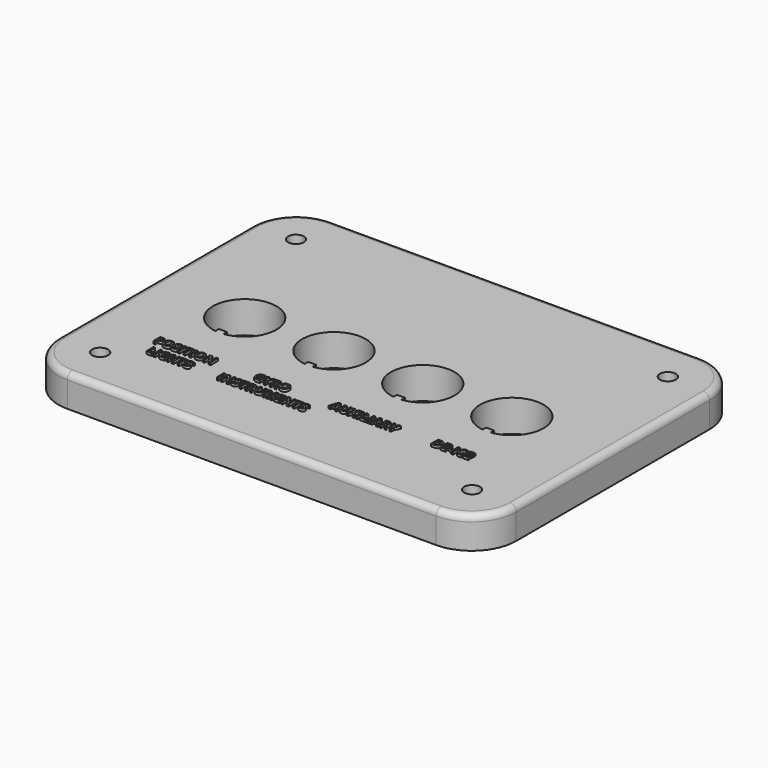
from build123d import *

# Parameters (mm, degrees)
F0_R         = 1.5875
F0_W         = 0.3738893229
F0_H         = 1.7629518229
F0_W_2       = 0.6474574653
F0_H_2       = 0.3013493924
F0_TEXT_SIZE = 2.4694444444
F1_DEPTH     = 6.35
F2_R         = 1.27
F3_DEPTH     = 0.508


# Not quite as in the source:
# - Text() gives the source's letters only with a copy of the font that has no kerning and outlines rounded to 1/6400 em; it was checked with that copy


with BuildPart() as f1:
    # F0 (on Top) → F1 (new body)
    with BuildSketch(Plane.XY):
        with BuildLine():
            ThreePointArc((-45.72, -22.8328104488), (-43.1161792847, -29.1189897335), (-36.83, -31.7228104488))
            Line((-36.83, -31.7228104488), (36.83, -31.7228104488))
            ThreePointArc((36.83, -31.7228104488), (43.1161792847, -29.1189897335), (45.72, -22.8328104488))
            Line((45.72, -22.8328104488), (45.72, 25.4271895512))
            ThreePointArc((45.72, 25.4271895512), (43.1161792847, 31.7133688359), (36.83, 34.3171895512))
            Line((36.83, 34.3171895512), (-36.83, 34.3171895512))
            ThreePointArc((-36.83, 34.3171895512), (-43.1161792847, 31.7133688359), (-45.72, 25.4271895512))
            Line((-45.72, 25.4271895512), (-45.72, -22.8328104488))
        make_face()
        with BuildLine():
            Line((33.655, -28.5478104488), (-33.655, -28.5478104488))
            ThreePointArc((-33.655, -28.5478104488), (-39.9411792847, -25.9439897335), (-42.545, -19.6578104488))
            Line((-42.545, -19.6578104488), (-42.545, 22.2521895512))
            ThreePointArc((-42.545, 22.2521895512), (-39.9411792847, 28.5383688359), (-33.655, 31.1421895512))
            Line((-33.655, 31.1421895512), (33.655, 31.1421895512))
            ThreePointArc((33.655, 31.1421895512), (39.9411792847, 28.5383688359), (42.545, 22.2521895512))
            Line((42.545, 22.2521895512), (42.545, -19.6578104488))
            ThreePointArc((42.545, -19.6578104488), (39.9411792847, -25.9439897335), (33.655, -28.5478104488))
        make_face(mode=Mode.SUBTRACT)
        with BuildLine():
            ThreePointArc((-42.545, -19.6578104488), (-39.9411792847, -25.9439897335), (-33.655, -28.5478104488))
            Line((-33.655, -28.5478104488), (33.655, -28.5478104488))
            ThreePointArc((33.655, -28.5478104488), (39.9411792847, -25.9439897335), (42.545, -19.6578104488))
            Line((42.545, -19.6578104488), (42.545, 22.2521895512))
            ThreePointArc((42.545, 22.2521895512), (39.9411792847, 28.5383688359), (33.655, 31.1421895512))
            Line((33.655, 31.1421895512), (-33.655, 31.1421895512))
            ThreePointArc((-33.655, 31.1421895512), (-39.9411792847, 28.5383688359), (-42.545, 22.2521895512))
            Line((-42.545, 22.2521895512), (-42.545, -19.6578104488))
        make_face()
        with Locations((-37.1475, -23.1503104488)):
            Circle(F0_R, mode=Mode.SUBTRACT)
        Polygon((-30.0736846576, -19.1064444444), (-31.1625553173, -19.1064444444), (-31.1625553173, -17.3434926215), (-30.7886659944, -17.3434926215), (-30.7886659944, -18.7977638889), (-30.0736846576, -18.7977638889), align=None, mode=Mode.SUBTRACT)
        with Locations((-29.5803745447, -18.224968533)):
            Rectangle(F0_W, F0_H, mode=Mode.SUBTRACT)
        with BuildLine():
            Line((-28.2806364805, -18.4277330729), (-28.2806364805, -18.1163515625))
            Line((-28.2806364805, -18.1163515625), (-27.5810891715, -18.1163515625))
            Line((-27.5810891715, -18.1163515625), (-27.5810891715, -19.0304318576))
            add(Edge.make_bspline(
                [(-27.5810891715, -19.0304318576), (-27.7512493277, -19.0859943576), (-27.9013452479, -19.1083736979)],
                knots=[0, 0, 0, 1, 1, 1], degree=2))
            add(Edge.make_bspline(
                [(-27.9013452479, -19.1083736979), (-28.051441168, -19.1307530382), (-28.2080965499, -19.1307530382)],
                knots=[0, 0, 0, 1, 1, 1], degree=2))
            add(Edge.make_bspline(
                [(-28.2080965499, -19.1307530382), (-28.607066168, -19.1307530382), (-28.8175477218, -18.896155816)],
                knots=[0, 0, 0, 1, 1, 1], degree=2))
            add(Edge.make_bspline(
                [(-28.8175477218, -18.896155816), (-29.0280292756, -18.6615585938), (-29.0280292756, -18.2224605035)],
                knots=[0, 0, 0, 1, 1, 1], degree=2))
            add(Edge.make_bspline(
                [(-29.0280292756, -18.2224605035), (-29.0280292756, -17.7957096354), (-28.7837857861, -17.5570609809)],
                knots=[0, 0, 0, 1, 1, 1], degree=2))
            add(Edge.make_bspline(
                [(-28.7837857861, -17.5570609809), (-28.5395422965, -17.3184123264), (-28.107003668, -17.3184123264)],
                knots=[0, 0, 0, 1, 1, 1], degree=2))
            add(Edge.make_bspline(
                [(-28.107003668, -17.3184123264), (-27.8353647791, -17.3184123264), (-27.5834042756, -17.4268363715)],
                knots=[0, 0, 0, 1, 1, 1], degree=2))
            Line((-27.5834042756, -17.4268363715), (-27.7076481993, -17.7258706597))
            add(Edge.make_bspline(
                [(-27.7076481993, -17.7258706597), (-27.9005735465, -17.6294079861), (-28.1093187722, -17.6294079861)],
                knots=[0, 0, 0, 1, 1, 1], degree=2))
            add(Edge.make_bspline(
                [(-28.1093187722, -17.6294079861), (-28.3516330083, -17.6294079861), (-28.4974845708, -17.7922369792)],
                knots=[0, 0, 0, 1, 1, 1], degree=2))
            add(Edge.make_bspline(
                [(-28.4974845708, -17.7922369792), (-28.6433361333, -17.9550659722), (-28.6433361333, -18.2297916667)],
                knots=[0, 0, 0, 1, 1, 1], degree=2))
            add(Edge.make_bspline(
                [(-28.6433361333, -18.2297916667), (-28.6433361333, -18.5168645833), (-28.5258445968, -18.6681180556)],
                knots=[0, 0, 0, 1, 1, 1], degree=2))
            add(Edge.make_bspline(
                [(-28.5258445968, -18.6681180556), (-28.4083530604, -18.8193715278), (-28.1841738069, -18.8193715278)],
                knots=[0, 0, 0, 1, 1, 1], degree=2))
            add(Edge.make_bspline(
                [(-28.1841738069, -18.8193715278), (-28.0668751958, -18.8193715278), (-27.9464897791, -18.7954487847)],
                knots=[0, 0, 0, 1, 1, 1], degree=2))
            Line((-27.9464897791, -18.7954487847), (-27.9464897791, -18.4277330729))
            Line((-27.9464897791, -18.4277330729), (-28.2806364805, -18.4277330729))
        make_face(mode=Mode.SUBTRACT)
        Polygon((-25.7170444666, -17.3434926215), (-25.7170444666, -19.1064444444), (-26.0897762374, -19.1064444444), (-26.0897762374, -18.345546875), (-26.7877801437, -18.345546875), (-26.7877801437, -19.1064444444), (-27.1616694666, -19.1064444444), (-27.1616694666, -17.3434926215), (-26.7877801437, -17.3434926215), (-26.7877801437, -18.0345512153), (-26.0897762374, -18.0345512153), (-26.0897762374, -17.3434926215), align=None, mode=Mode.SUBTRACT)
        Polygon((-24.5919038416, -17.6544882813), (-24.5919038416, -19.1064444444), (-24.9657931645, -19.1064444444), (-24.9657931645, -17.6544882813), (-25.4446338763, -17.6544882813), (-25.4446338763, -17.3434926215), (-24.1134489805, -17.3434926215), (-24.1134489805, -17.6544882813), align=None, mode=Mode.SUBTRACT)
        with BuildLine():
            add(Edge.make_bspline(
                [(-22.8931961593, -18.3256755642), (-22.8015566194, -18.4443246528), (-22.8015566194, -18.6167999132)],
                knots=[0, 0, 0, 1, 1, 1], degree=2))
            add(Edge.make_bspline(
                [(-22.8015566194, -18.6167999132), (-22.8015566194, -18.8556414931), (-22.9734531038, -18.9931972656)],
                knots=[0, 0, 0, 1, 1, 1], degree=2))
            add(Edge.make_bspline(
                [(-22.9734531038, -18.9931972656), (-23.1453495881, -19.1307530382), (-23.4513291888, -19.1307530382)],
                knots=[0, 0, 0, 1, 1, 1], degree=2))
            add(Edge.make_bspline(
                [(-23.4513291888, -19.1307530382), (-23.7337718972, -19.1307530382), (-23.9506199874, -19.0242582465)],
                knots=[0, 0, 0, 1, 1, 1], degree=2))
            Line((-23.9506199874, -19.0242582465), (-23.9506199874, -18.6769926215))
            add(Edge.make_bspline(
                [(-23.9506199874, -18.6769926215), (-23.7723569666, -18.7568637153), (-23.648691819, -18.7892751736)],
                knots=[0, 0, 0, 1, 1, 1], degree=2))
            add(Edge.make_bspline(
                [(-23.648691819, -18.7892751736), (-23.5250266715, -18.8216866319), (-23.4223903868, -18.8216866319)],
                knots=[0, 0, 0, 1, 1, 1], degree=2))
            add(Edge.make_bspline(
                [(-23.4223903868, -18.8216866319), (-23.2996898659, -18.8216866319), (-23.2339023225, -18.7748057726)],
                knots=[0, 0, 0, 1, 1, 1], degree=2))
            add(Edge.make_bspline(
                [(-23.2339023225, -18.7748057726), (-23.1681147791, -18.7279249132), (-23.1681147791, -18.6349348958)],
                knots=[0, 0, 0, 1, 1, 1], degree=2))
            add(Edge.make_bspline(
                [(-23.1681147791, -18.6349348958), (-23.1681147791, -18.5832309028), (-23.1970535812, -18.5427165799)],
                knots=[0, 0, 0, 1, 1, 1], degree=2))
            add(Edge.make_bspline(
                [(-23.1970535812, -18.5427165799), (-23.2259923833, -18.5022022569), (-23.2821336593, -18.4649676649)],
                knots=[0, 0, 0, 1, 1, 1], degree=2))
            add(Edge.make_bspline(
                [(-23.2821336593, -18.4649676649), (-23.3382749354, -18.4277330729), (-23.5107501958, -18.345546875)],
                knots=[0, 0, 0, 1, 1, 1], degree=2))
            add(Edge.make_bspline(
                [(-23.5107501958, -18.345546875), (-23.6720357861, -18.2695342882), (-23.7528715065, -18.1996953125)],
                knots=[0, 0, 0, 1, 1, 1], degree=2))
            add(Edge.make_bspline(
                [(-23.7528715065, -18.1996953125), (-23.833707227, -18.1298563368), (-23.8819385638, -18.0368663194)],
                knots=[0, 0, 0, 1, 1, 1], degree=2))
            add(Edge.make_bspline(
                [(-23.8819385638, -18.0368663194), (-23.9301699006, -17.9438763021), (-23.9301699006, -17.8200182292)],
                knots=[0, 0, 0, 1, 1, 1], degree=2))
            add(Edge.make_bspline(
                [(-23.9301699006, -17.8200182292), (-23.9301699006, -17.5858068576), (-23.7715852652, -17.452109592)],
                knots=[0, 0, 0, 1, 1, 1], degree=2))
            add(Edge.make_bspline(
                [(-23.7715852652, -17.452109592), (-23.6130006298, -17.3184123264), (-23.3332588763, -17.3184123264)],
                knots=[0, 0, 0, 1, 1, 1], degree=2))
            add(Edge.make_bspline(
                [(-23.3332588763, -17.3184123264), (-23.1958960291, -17.3184123264), (-23.0710733295, -17.3508237847)],
                knots=[0, 0, 0, 1, 1, 1], degree=2))
            add(Edge.make_bspline(
                [(-23.0710733295, -17.3508237847), (-22.9462506298, -17.3832352431), (-22.8100453347, -17.4422703993)],
                knots=[0, 0, 0, 1, 1, 1], degree=2))
            Line((-22.8100453347, -17.4422703993), (-22.9304307513, -17.7332018229))
            add(Edge.make_bspline(
                [(-22.9304307513, -17.7332018229), (-23.0716521055, -17.6753242188), (-23.1638704215, -17.6523661024)],
                knots=[0, 0, 0, 1, 1, 1], degree=2))
            add(Edge.make_bspline(
                [(-23.1638704215, -17.6523661024), (-23.2560887374, -17.6294079861), (-23.3452202479, -17.6294079861)],
                knots=[0, 0, 0, 1, 1, 1], degree=2))
            add(Edge.make_bspline(
                [(-23.3452202479, -17.6294079861), (-23.4513291888, -17.6294079861), (-23.5080492409, -17.678796875)],
                knots=[0, 0, 0, 1, 1, 1], degree=2))
            add(Edge.make_bspline(
                [(-23.5080492409, -17.678796875), (-23.564769293, -17.7281857639), (-23.564769293, -17.8076710069)],
                knots=[0, 0, 0, 1, 1, 1], degree=2))
            add(Edge.make_bspline(
                [(-23.564769293, -17.8076710069), (-23.564769293, -17.8570598958), (-23.5418111767, -17.8939086372)],
                knots=[0, 0, 0, 1, 1, 1], degree=2))
            add(Edge.make_bspline(
                [(-23.5418111767, -17.8939086372), (-23.5188530604, -17.9307573785), (-23.4688853954, -17.9650980903)],
                knots=[0, 0, 0, 1, 1, 1], degree=2))
            add(Edge.make_bspline(
                [(-23.4688853954, -17.9650980903), (-23.4189177305, -17.9994388021), (-23.2321659944, -18.0885703125)],
                knots=[0, 0, 0, 1, 1, 1], degree=2))
            add(Edge.make_bspline(
                [(-23.2321659944, -18.0885703125), (-22.9848356993, -18.2070264757), (-22.8931961593, -18.3256755642)],
                knots=[0, 0, 0, 1, 1, 1], degree=2))
        make_face(mode=Mode.SUBTRACT)
        with Locations((-16.8888935736, -18.224968533)):
            Rectangle(F0_W, F0_H, mode=Mode.SUBTRACT)
        with BuildLine():
            Line((-14.694367749, -17.3434926215), (-14.694367749, -19.1064444444))
            Line((-14.694367749, -19.1064444444), (-15.1693499538, -19.1064444444))
            Line((-15.1693499538, -19.1064444444), (-15.9364211344, -17.7729444444))
            Line((-15.9364211344, -17.7729444444), (-15.9472249538, -17.7729444444))
            add(Edge.make_bspline(
                [(-15.9472249538, -17.7729444444), (-15.9240739122, -18.1259978299), (-15.9240739122, -18.2768654514)],
                knots=[0, 0, 0, 1, 1, 1], degree=2))
            Line((-15.9240739122, -18.2768654514), (-15.9240739122, -19.1064444444))
            Line((-15.9240739122, -19.1064444444), (-16.2582206136, -19.1064444444))
            Line((-16.2582206136, -19.1064444444), (-16.2582206136, -17.3434926215))
            Line((-16.2582206136, -17.3434926215), (-15.7867110649, -17.3434926215))
            Line((-15.7867110649, -17.3434926215), (-15.0211832872, -18.6638736979))
            Line((-15.0211832872, -18.6638736979), (-15.0126945719, -18.6638736979))
            add(Edge.make_bspline(
                [(-15.0126945719, -18.6638736979), (-15.0308295545, -18.3200807292), (-15.0308295545, -18.1780876736)],
                knots=[0, 0, 0, 1, 1, 1], degree=2))
            Line((-15.0308295545, -18.1780876736), (-15.0308295545, -17.3434926215))
            Line((-15.0308295545, -17.3434926215), (-14.694367749, -17.3434926215))
        make_face(mode=Mode.SUBTRACT)
        with BuildLine():
            add(Edge.make_bspline(
                [(-13.3016396674, -18.3256755642), (-13.2100001274, -18.4443246528), (-13.2100001274, -18.6167999132)],
                knots=[0, 0, 0, 1, 1, 1], degree=2))
            add(Edge.make_bspline(
                [(-13.2100001274, -18.6167999132), (-13.2100001274, -18.8556414931), (-13.3818966118, -18.9931972656)],
                knots=[0, 0, 0, 1, 1, 1], degree=2))
            add(Edge.make_bspline(
                [(-13.3818966118, -18.9931972656), (-13.5537930962, -19.1307530382), (-13.8597726969, -19.1307530382)],
                knots=[0, 0, 0, 1, 1, 1], degree=2))
            add(Edge.make_bspline(
                [(-13.8597726969, -19.1307530382), (-14.1422154052, -19.1307530382), (-14.3590634955, -19.0242582465)],
                knots=[0, 0, 0, 1, 1, 1], degree=2))
            Line((-14.3590634955, -19.0242582465), (-14.3590634955, -18.6769926215))
            add(Edge.make_bspline(
                [(-14.3590634955, -18.6769926215), (-14.1808004747, -18.7568637153), (-14.0571353271, -18.7892751736)],
                knots=[0, 0, 0, 1, 1, 1], degree=2))
            add(Edge.make_bspline(
                [(-14.0571353271, -18.7892751736), (-13.9334701795, -18.8216866319), (-13.8308338948, -18.8216866319)],
                knots=[0, 0, 0, 1, 1, 1], degree=2))
            add(Edge.make_bspline(
                [(-13.8308338948, -18.8216866319), (-13.708133374, -18.8216866319), (-13.6423458306, -18.7748057726)],
                knots=[0, 0, 0, 1, 1, 1], degree=2))
            add(Edge.make_bspline(
                [(-13.6423458306, -18.7748057726), (-13.5765582872, -18.7279249132), (-13.5765582872, -18.6349348958)],
                knots=[0, 0, 0, 1, 1, 1], degree=2))
            add(Edge.make_bspline(
                [(-13.5765582872, -18.6349348958), (-13.5765582872, -18.5832309028), (-13.6054970893, -18.5427165799)],
                knots=[0, 0, 0, 1, 1, 1], degree=2))
            add(Edge.make_bspline(
                [(-13.6054970893, -18.5427165799), (-13.6344358913, -18.5022022569), (-13.6905771674, -18.4649676649)],
                knots=[0, 0, 0, 1, 1, 1], degree=2))
            add(Edge.make_bspline(
                [(-13.6905771674, -18.4649676649), (-13.7467184434, -18.4277330729), (-13.9191937038, -18.345546875)],
                knots=[0, 0, 0, 1, 1, 1], degree=2))
            add(Edge.make_bspline(
                [(-13.9191937038, -18.345546875), (-14.0804792941, -18.2695342882), (-14.1613150146, -18.1996953125)],
                knots=[0, 0, 0, 1, 1, 1], degree=2))
            add(Edge.make_bspline(
                [(-14.1613150146, -18.1996953125), (-14.2421507351, -18.1298563368), (-14.2903820719, -18.0368663194)],
                knots=[0, 0, 0, 1, 1, 1], degree=2))
            add(Edge.make_bspline(
                [(-14.2903820719, -18.0368663194), (-14.3386134087, -17.9438763021), (-14.3386134087, -17.8200182292)],
                knots=[0, 0, 0, 1, 1, 1], degree=2))
            add(Edge.make_bspline(
                [(-14.3386134087, -17.8200182292), (-14.3386134087, -17.5858068576), (-14.1800287733, -17.452109592)],
                knots=[0, 0, 0, 1, 1, 1], degree=2))
            add(Edge.make_bspline(
                [(-14.1800287733, -17.452109592), (-14.0214441379, -17.3184123264), (-13.7417023844, -17.3184123264)],
                knots=[0, 0, 0, 1, 1, 1], degree=2))
            add(Edge.make_bspline(
                [(-13.7417023844, -17.3184123264), (-13.6043395372, -17.3184123264), (-13.4795168375, -17.3508237847)],
                knots=[0, 0, 0, 1, 1, 1], degree=2))
            add(Edge.make_bspline(
                [(-13.4795168375, -17.3508237847), (-13.3546941379, -17.3832352431), (-13.2184888427, -17.4422703993)],
                knots=[0, 0, 0, 1, 1, 1], degree=2))
            Line((-13.2184888427, -17.4422703993), (-13.3388742594, -17.7332018229))
            add(Edge.make_bspline(
                [(-13.3388742594, -17.7332018229), (-13.4800956136, -17.6753242188), (-13.5723139295, -17.6523661024)],
                knots=[0, 0, 0, 1, 1, 1], degree=2))
            add(Edge.make_bspline(
                [(-13.5723139295, -17.6523661024), (-13.6645322455, -17.6294079861), (-13.7536637559, -17.6294079861)],
                knots=[0, 0, 0, 1, 1, 1], degree=2))
            add(Edge.make_bspline(
                [(-13.7536637559, -17.6294079861), (-13.8597726969, -17.6294079861), (-13.916492749, -17.678796875)],
                knots=[0, 0, 0, 1, 1, 1], degree=2))
            add(Edge.make_bspline(
                [(-13.916492749, -17.678796875), (-13.9732128011, -17.7281857639), (-13.9732128011, -17.8076710069)],
                knots=[0, 0, 0, 1, 1, 1], degree=2))
            add(Edge.make_bspline(
                [(-13.9732128011, -17.8076710069), (-13.9732128011, -17.8570598958), (-13.9502546847, -17.8939086372)],
                knots=[0, 0, 0, 1, 1, 1], degree=2))
            add(Edge.make_bspline(
                [(-13.9502546847, -17.8939086372), (-13.9272965684, -17.9307573785), (-13.8773289035, -17.9650980903)],
                knots=[0, 0, 0, 1, 1, 1], degree=2))
            add(Edge.make_bspline(
                [(-13.8773289035, -17.9650980903), (-13.8273612386, -17.9994388021), (-13.6406095024, -18.0885703125)],
                knots=[0, 0, 0, 1, 1, 1], degree=2))
            add(Edge.make_bspline(
                [(-13.6406095024, -18.0885703125), (-13.3932792073, -18.2070264757), (-13.3016396674, -18.3256755642)],
                knots=[0, 0, 0, 1, 1, 1], degree=2))
        make_face(mode=Mode.SUBTRACT)
        Polygon((-12.2102609781, -17.6544882813), (-12.2102609781, -19.1064444444), (-12.5841503011, -19.1064444444), (-12.5841503011, -17.6544882813), (-13.0629910129, -17.6544882813), (-13.0629910129, -17.3434926215), (-11.731806117, -17.3434926215), (-11.731806117, -17.6544882813), align=None, mode=Mode.SUBTRACT)
        with BuildLine():
            Line((-10.8879506483, -18.4300481771), (-11.0866637559, -18.4300481771))
            Line((-11.0866637559, -18.4300481771), (-11.0866637559, -19.1064444444))
            Line((-11.0866637559, -19.1064444444), (-11.4605530788, -19.1064444444))
            Line((-11.4605530788, -19.1064444444), (-11.4605530788, -17.3434926215))
            Line((-11.4605530788, -17.3434926215), (-10.9469858045, -17.3434926215))
            add(Edge.make_bspline(
                [(-10.9469858045, -17.3434926215), (-10.5873729573, -17.3434926215), (-10.4150906222, -17.4742960069)],
                knots=[0, 0, 0, 1, 1, 1], degree=2))
            add(Edge.make_bspline(
                [(-10.4150906222, -17.4742960069), (-10.2428082872, -17.6050993924), (-10.2428082872, -17.8717222222)],
                knots=[0, 0, 0, 1, 1, 1], degree=2))
            add(Edge.make_bspline(
                [(-10.2428082872, -17.8717222222), (-10.2428082872, -18.0272200521), (-10.328274216, -18.1483771701)],
                knots=[0, 0, 0, 1, 1, 1], degree=2))
            add(Edge.make_bspline(
                [(-10.328274216, -18.1483771701), (-10.4137401448, -18.2695342882), (-10.5707813774, -18.3382157118)],
                knots=[0, 0, 0, 1, 1, 1], degree=2))
            add(Edge.make_bspline(
                [(-10.5707813774, -18.3382157118), (-10.1725834608, -18.9328116319), (-10.0521980441, -19.1064444444)],
                knots=[0, 0, 0, 1, 1, 1], degree=2))
            Line((-10.0521980441, -19.1064444444), (-10.4669875406, -19.1064444444))
            Line((-10.4669875406, -19.1064444444), (-10.8879506483, -18.4300481771))
        make_face(mode=Mode.SUBTRACT)
        with BuildLine():
            Line((-8.768086933, -17.3434926215), (-8.3953551622, -17.3434926215))
            Line((-8.3953551622, -17.3434926215), (-8.3953551622, -18.4840672743))
            add(Edge.make_bspline(
                [(-8.3953551622, -18.4840672743), (-8.3953551622, -18.6796935764), (-8.4827503445, -18.826702691)],
                knots=[0, 0, 0, 1, 1, 1], degree=2))
            add(Edge.make_bspline(
                [(-8.4827503445, -18.826702691), (-8.5701455268, -18.9737118056), (-8.7354825493, -19.0522324219)],
                knots=[0, 0, 0, 1, 1, 1], degree=2))
            add(Edge.make_bspline(
                [(-8.7354825493, -19.0522324219), (-8.9008195719, -19.1307530382), (-9.1261563774, -19.1307530382)],
                knots=[0, 0, 0, 1, 1, 1], degree=2))
            add(Edge.make_bspline(
                [(-9.1261563774, -19.1307530382), (-9.4660908393, -19.1307530382), (-9.6541930528, -18.9563485243)],
                knots=[0, 0, 0, 1, 1, 1], degree=2))
            add(Edge.make_bspline(
                [(-9.6541930528, -18.9563485243), (-9.8422952663, -18.7819440104), (-9.8422952663, -18.479437066)],
                knots=[0, 0, 0, 1, 1, 1], degree=2))
            Line((-9.8422952663, -18.479437066), (-9.8422952663, -17.3434926215))
            Line((-9.8422952663, -17.3434926215), (-9.4699493462, -17.3434926215))
            Line((-9.4699493462, -17.3434926215), (-9.4699493462, -18.4227170139))
            add(Edge.make_bspline(
                [(-9.4699493462, -18.4227170139), (-9.4699493462, -18.6264461806), (-9.3879560736, -18.7217513021)],
                knots=[0, 0, 0, 1, 1, 1], degree=2))
            add(Edge.make_bspline(
                [(-9.3879560736, -18.7217513021), (-9.3059628011, -18.8170564236), (-9.1165101101, -18.8170564236)],
                knots=[0, 0, 0, 1, 1, 1], degree=2))
            add(Edge.make_bspline(
                [(-9.1165101101, -18.8170564236), (-8.9332310302, -18.8170564236), (-8.8506589816, -18.721172526)],
                knots=[0, 0, 0, 1, 1, 1], degree=2))
            add(Edge.make_bspline(
                [(-8.8506589816, -18.721172526), (-8.768086933, -18.6252886285), (-8.768086933, -18.4204019097)],
                knots=[0, 0, 0, 1, 1, 1], degree=2))
            Line((-8.768086933, -18.4204019097), (-8.768086933, -17.3434926215))
        make_face(mode=Mode.SUBTRACT)
        with BuildLine():
            Line((-6.8747175754, -19.1064444444), (-7.217352992, -19.1064444444))
            Line((-7.217352992, -19.1064444444), (-7.6417887559, -17.7235555556))
            Line((-7.6417887559, -17.7235555556), (-7.6525925754, -17.7235555556))
            add(Edge.make_bspline(
                [(-7.6525925754, -17.7235555556), (-7.6294415337, -18.1452903646), (-7.6294415337, -18.2865117188)],
                knots=[0, 0, 0, 1, 1, 1], degree=2))
            Line((-7.6294415337, -18.2865117188), (-7.6294415337, -19.1064444444))
            Line((-7.6294415337, -19.1064444444), (-7.9635882351, -19.1064444444))
            Line((-7.9635882351, -19.1064444444), (-7.9635882351, -17.3434926215))
            Line((-7.9635882351, -17.3434926215), (-7.4546511691, -17.3434926215))
            Line((-7.4546511691, -17.3434926215), (-7.0375465684, -18.6916549479))
            Line((-7.0375465684, -18.6916549479), (-7.0302154052, -18.6916549479))
            Line((-7.0302154052, -18.6916549479), (-6.5876446587, -17.3434926215))
            Line((-6.5876446587, -17.3434926215), (-6.0790934434, -17.3434926215))
            Line((-6.0790934434, -17.3434926215), (-6.0790934434, -19.1064444444))
            Line((-6.0790934434, -19.1064444444), (-6.4275166205, -19.1064444444))
            Line((-6.4275166205, -19.1064444444), (-6.4275166205, -18.2718493924))
            add(Edge.make_bspline(
                [(-6.4275166205, -18.2718493924), (-6.4275166205, -18.2128142361), (-6.425587367, -18.1356440972)],
                knots=[0, 0, 0, 1, 1, 1], degree=2))
            add(Edge.make_bspline(
                [(-6.425587367, -18.1356440972), (-6.4236581136, -18.0584739583), (-6.4093816379, -17.7258706597)],
                knots=[0, 0, 0, 1, 1, 1], degree=2))
            Line((-6.4093816379, -17.7258706597), (-6.4201854573, -17.7258706597))
            Line((-6.4201854573, -17.7258706597), (-6.8747175754, -19.1064444444))
        make_face(mode=Mode.SUBTRACT)
        Polygon((-4.6201919677, -18.7977638889), (-4.6201919677, -19.1064444444), (-5.6353651448, -19.1064444444), (-5.6353651448, -17.3434926215), (-4.6201919677, -17.3434926215), (-4.6201919677, -17.6498580729), (-5.2614758219, -17.6498580729), (-5.2614758219, -18.0368663194), (-4.6645647976, -18.0368663194), (-4.6645647976, -18.3432317708), (-5.2614758219, -18.3432317708), (-5.2614758219, -18.7977638889), align=None, mode=Mode.SUBTRACT)
        with BuildLine():
            Line((-2.6886233913, -17.3434926215), (-2.6886233913, -19.1064444444))
            Line((-2.6886233913, -19.1064444444), (-3.1636055962, -19.1064444444))
            Line((-3.1636055962, -19.1064444444), (-3.9306767768, -17.7729444444))
            Line((-3.9306767768, -17.7729444444), (-3.9414805962, -17.7729444444))
            add(Edge.make_bspline(
                [(-3.9414805962, -17.7729444444), (-3.9183295545, -18.1259978299), (-3.9183295545, -18.2768654514)],
                knots=[0, 0, 0, 1, 1, 1], degree=2))
            Line((-3.9183295545, -18.2768654514), (-3.9183295545, -19.1064444444))
            Line((-3.9183295545, -19.1064444444), (-4.2524762559, -19.1064444444))
            Line((-4.2524762559, -19.1064444444), (-4.2524762559, -17.3434926215))
            Line((-4.2524762559, -17.3434926215), (-3.7809667073, -17.3434926215))
            Line((-3.7809667073, -17.3434926215), (-3.0154389295, -18.6638736979))
            Line((-3.0154389295, -18.6638736979), (-3.0069502143, -18.6638736979))
            add(Edge.make_bspline(
                [(-3.0069502143, -18.6638736979), (-3.0250851969, -18.3200807292), (-3.0250851969, -18.1780876736)],
                knots=[0, 0, 0, 1, 1, 1], degree=2))
            Line((-3.0250851969, -18.1780876736), (-3.0250851969, -17.3434926215))
            Line((-3.0250851969, -17.3434926215), (-2.6886233913, -17.3434926215))
        make_face(mode=Mode.SUBTRACT)
        Polygon((-1.5646403184, -17.6544882813), (-1.5646403184, -19.1064444444), (-1.9385296413, -19.1064444444), (-1.9385296413, -17.6544882813), (-2.4173703531, -17.6544882813), (-2.4173703531, -17.3434926215), (-1.0861854573, -17.3434926215), (-1.0861854573, -17.6544882813), align=None, mode=Mode.SUBTRACT)
        with BuildLine():
            add(Edge.make_bspline(
                [(0.1340673639, -18.3256755642), (0.2257069038, -18.4443246528), (0.2257069038, -18.6167999132)],
                knots=[0, 0, 0, 1, 1, 1], degree=2))
            add(Edge.make_bspline(
                [(0.2257069038, -18.6167999132), (0.2257069038, -18.8556414931), (0.0538104194, -18.9931972656)],
                knots=[0, 0, 0, 1, 1, 1], degree=2))
            add(Edge.make_bspline(
                [(0.0538104194, -18.9931972656), (-0.1180860649, -19.1307530382), (-0.4240656656, -19.1307530382)],
                knots=[0, 0, 0, 1, 1, 1], degree=2))
            add(Edge.make_bspline(
                [(-0.4240656656, -19.1307530382), (-0.706508374, -19.1307530382), (-0.9233564643, -19.0242582465)],
                knots=[0, 0, 0, 1, 1, 1], degree=2))
            Line((-0.9233564643, -19.0242582465), (-0.9233564643, -18.6769926215))
            add(Edge.make_bspline(
                [(-0.9233564643, -18.6769926215), (-0.7450934434, -18.7568637153), (-0.6214282959, -18.7892751736)],
                knots=[0, 0, 0, 1, 1, 1], degree=2))
            add(Edge.make_bspline(
                [(-0.6214282959, -18.7892751736), (-0.4977631483, -18.8216866319), (-0.3951268636, -18.8216866319)],
                knots=[0, 0, 0, 1, 1, 1], degree=2))
            add(Edge.make_bspline(
                [(-0.3951268636, -18.8216866319), (-0.2724263427, -18.8216866319), (-0.2066387993, -18.7748057726)],
                knots=[0, 0, 0, 1, 1, 1], degree=2))
            add(Edge.make_bspline(
                [(-0.2066387993, -18.7748057726), (-0.1408512559, -18.7279249132), (-0.1408512559, -18.6349348958)],
                knots=[0, 0, 0, 1, 1, 1], degree=2))
            add(Edge.make_bspline(
                [(-0.1408512559, -18.6349348958), (-0.1408512559, -18.5832309028), (-0.169790058, -18.5427165799)],
                knots=[0, 0, 0, 1, 1, 1], degree=2))
            add(Edge.make_bspline(
                [(-0.169790058, -18.5427165799), (-0.1987288601, -18.5022022569), (-0.2548701361, -18.4649676649)],
                knots=[0, 0, 0, 1, 1, 1], degree=2))
            add(Edge.make_bspline(
                [(-0.2548701361, -18.4649676649), (-0.3110114122, -18.4277330729), (-0.4834866726, -18.345546875)],
                knots=[0, 0, 0, 1, 1, 1], degree=2))
            add(Edge.make_bspline(
                [(-0.4834866726, -18.345546875), (-0.6447722629, -18.2695342882), (-0.7256079834, -18.1996953125)],
                knots=[0, 0, 0, 1, 1, 1], degree=2))
            add(Edge.make_bspline(
                [(-0.7256079834, -18.1996953125), (-0.8064437038, -18.1298563368), (-0.8546750406, -18.0368663194)],
                knots=[0, 0, 0, 1, 1, 1], degree=2))
            add(Edge.make_bspline(
                [(-0.8546750406, -18.0368663194), (-0.9029063774, -17.9438763021), (-0.9029063774, -17.8200182292)],
                knots=[0, 0, 0, 1, 1, 1], degree=2))
            add(Edge.make_bspline(
                [(-0.9029063774, -17.8200182292), (-0.9029063774, -17.5858068576), (-0.744321742, -17.452109592)],
                knots=[0, 0, 0, 1, 1, 1], degree=2))
            add(Edge.make_bspline(
                [(-0.744321742, -17.452109592), (-0.5857371066, -17.3184123264), (-0.3059953531, -17.3184123264)],
                knots=[0, 0, 0, 1, 1, 1], degree=2))
            add(Edge.make_bspline(
                [(-0.3059953531, -17.3184123264), (-0.1686325059, -17.3184123264), (-0.0438098063, -17.3508237847)],
                knots=[0, 0, 0, 1, 1, 1], degree=2))
            add(Edge.make_bspline(
                [(-0.0438098063, -17.3508237847), (0.0810128934, -17.3832352431), (0.2172181885, -17.4422703993)],
                knots=[0, 0, 0, 1, 1, 1], degree=2))
            Line((0.2172181885, -17.4422703993), (0.0968327719, -17.7332018229))
            add(Edge.make_bspline(
                [(0.0968327719, -17.7332018229), (-0.0443885823, -17.6753242188), (-0.1366068983, -17.6523661024)],
                knots=[0, 0, 0, 1, 1, 1], degree=2))
            add(Edge.make_bspline(
                [(-0.1366068983, -17.6523661024), (-0.2288252143, -17.6294079861), (-0.3179567247, -17.6294079861)],
                knots=[0, 0, 0, 1, 1, 1], degree=2))
            add(Edge.make_bspline(
                [(-0.3179567247, -17.6294079861), (-0.4240656656, -17.6294079861), (-0.4807857177, -17.678796875)],
                knots=[0, 0, 0, 1, 1, 1], degree=2))
            add(Edge.make_bspline(
                [(-0.4807857177, -17.678796875), (-0.5375057698, -17.7281857639), (-0.5375057698, -17.8076710069)],
                knots=[0, 0, 0, 1, 1, 1], degree=2))
            add(Edge.make_bspline(
                [(-0.5375057698, -17.8076710069), (-0.5375057698, -17.8570598958), (-0.5145476535, -17.8939086372)],
                knots=[0, 0, 0, 1, 1, 1], degree=2))
            add(Edge.make_bspline(
                [(-0.5145476535, -17.8939086372), (-0.4915895372, -17.9307573785), (-0.4416218722, -17.9650980903)],
                knots=[0, 0, 0, 1, 1, 1], degree=2))
            add(Edge.make_bspline(
                [(-0.4416218722, -17.9650980903), (-0.3916542073, -17.9994388021), (-0.2049024712, -18.0885703125)],
                knots=[0, 0, 0, 1, 1, 1], degree=2))
            add(Edge.make_bspline(
                [(-0.2049024712, -18.0885703125), (0.0424278239, -18.2070264757), (0.1340673639, -18.3256755642)],
                knots=[0, 0, 0, 1, 1, 1], degree=2))
        make_face(mode=Mode.SUBTRACT)
        with BuildLine():
            add(Edge.make_bspline(
                [(-31.3950303607, -14.1231827257), (-31.2281499354, -14.2613172743), (-31.2281499354, -14.5348854167)],
                knots=[0, 0, 0, 1, 1, 1], degree=2))
            add(Edge.make_bspline(
                [(-31.2281499354, -14.5348854167), (-31.2281499354, -14.8196432292), (-31.4060271055, -14.9703179253)],
                knots=[0, 0, 0, 1, 1, 1], degree=2))
            add(Edge.make_bspline(
                [(-31.4060271055, -14.9703179253), (-31.5839042756, -15.1209926215), (-31.9118773659, -15.1209926215)],
                knots=[0, 0, 0, 1, 1, 1], degree=2))
            Line((-31.9118773659, -15.1209926215), (-32.0720054041, -15.1209926215))
            Line((-32.0720054041, -15.1209926215), (-32.0720054041, -15.748))
            Line((-32.0720054041, -15.748), (-32.445894727, -15.748))
            Line((-32.445894727, -15.748), (-32.445894727, -13.9850481771))
            Line((-32.445894727, -13.9850481771), (-31.8829385638, -13.9850481771))
            add(Edge.make_bspline(
                [(-31.8829385638, -13.9850481771), (-31.5619107861, -13.9850481771), (-31.3950303607, -14.1231827257)],
                knots=[0, 0, 0, 1, 1, 1], degree=2))
        make_face(mode=Mode.SUBTRACT)
        with BuildLine():
            add(Edge.make_bspline(
                [(-29.5103426437, -14.1912853733), (-29.2950379562, -14.4253038194), (-29.2950379562, -14.864016059)],
                knots=[0, 0, 0, 1, 1, 1], degree=2))
            add(Edge.make_bspline(
                [(-29.2950379562, -14.864016059), (-29.2950379562, -15.3019565972), (-29.5120789718, -15.5371325955)],
                knots=[0, 0, 0, 1, 1, 1], degree=2))
            add(Edge.make_bspline(
                [(-29.5120789718, -15.5371325955), (-29.7291199874, -15.7723085938), (-30.1342632166, -15.7723085938)],
                knots=[0, 0, 0, 1, 1, 1], degree=2))
            add(Edge.make_bspline(
                [(-30.1342632166, -15.7723085938), (-30.5394064458, -15.7723085938), (-30.7564474614, -15.5371325955)],
                knots=[0, 0, 0, 1, 1, 1], degree=2))
            add(Edge.make_bspline(
                [(-30.7564474614, -15.5371325955), (-30.973488477, -15.3019565972), (-30.973488477, -14.8617009549)],
                knots=[0, 0, 0, 1, 1, 1], degree=2))
            add(Edge.make_bspline(
                [(-30.973488477, -14.8617009549), (-30.973488477, -14.4214453125), (-30.7558686854, -14.1893561198)],
                knots=[0, 0, 0, 1, 1, 1], degree=2))
            add(Edge.make_bspline(
                [(-30.7558686854, -14.1893561198), (-30.5382488937, -13.9572669271), (-30.1319481124, -13.9572669271)],
                knots=[0, 0, 0, 1, 1, 1], degree=2))
            add(Edge.make_bspline(
                [(-30.1319481124, -13.9572669271), (-29.7256473312, -13.9572669271), (-29.5103426437, -14.1912853733)],
                knots=[0, 0, 0, 1, 1, 1], degree=2))
        make_face(mode=Mode.SUBTRACT)
        with BuildLine():
            add(Edge.make_bspline(
                [(-27.9806375656, -14.9672311198), (-27.8889980256, -15.0858802083), (-27.8889980256, -15.2583554688)],
                knots=[0, 0, 0, 1, 1, 1], degree=2))
            add(Edge.make_bspline(
                [(-27.8889980256, -15.2583554688), (-27.8889980256, -15.4971970486), (-28.06089451, -15.6347528212)],
                knots=[0, 0, 0, 1, 1, 1], degree=2))
            add(Edge.make_bspline(
                [(-28.06089451, -15.6347528212), (-28.2327909944, -15.7723085938), (-28.5387705951, -15.7723085938)],
                knots=[0, 0, 0, 1, 1, 1], degree=2))
            add(Edge.make_bspline(
                [(-28.5387705951, -15.7723085938), (-28.8212133034, -15.7723085938), (-29.0380613937, -15.6658138021)],
                knots=[0, 0, 0, 1, 1, 1], degree=2))
            Line((-29.0380613937, -15.6658138021), (-29.0380613937, -15.3185481771))
            add(Edge.make_bspline(
                [(-29.0380613937, -15.3185481771), (-28.8597983729, -15.3984192708), (-28.7361332253, -15.4308307292)],
                knots=[0, 0, 0, 1, 1, 1], degree=2))
            add(Edge.make_bspline(
                [(-28.7361332253, -15.4308307292), (-28.6124680777, -15.4632421875), (-28.509831793, -15.4632421875)],
                knots=[0, 0, 0, 1, 1, 1], degree=2))
            add(Edge.make_bspline(
                [(-28.509831793, -15.4632421875), (-28.3871312722, -15.4632421875), (-28.3213437288, -15.4163613281)],
                knots=[0, 0, 0, 1, 1, 1], degree=2))
            add(Edge.make_bspline(
                [(-28.3213437288, -15.4163613281), (-28.2555561854, -15.3694804688), (-28.2555561854, -15.2764904514)],
                knots=[0, 0, 0, 1, 1, 1], degree=2))
            add(Edge.make_bspline(
                [(-28.2555561854, -15.2764904514), (-28.2555561854, -15.2247864583), (-28.2844949874, -15.1842721354)],
                knots=[0, 0, 0, 1, 1, 1], degree=2))
            add(Edge.make_bspline(
                [(-28.2844949874, -15.1842721354), (-28.3134337895, -15.1437578125), (-28.3695750656, -15.1065232205)],
                knots=[0, 0, 0, 1, 1, 1], degree=2))
            add(Edge.make_bspline(
                [(-28.3695750656, -15.1065232205), (-28.4257163416, -15.0692886285), (-28.598191602, -14.9871024306)],
                knots=[0, 0, 0, 1, 1, 1], degree=2))
            add(Edge.make_bspline(
                [(-28.598191602, -14.9871024306), (-28.7594771923, -14.9110898438), (-28.8403129128, -14.8412508681)],
                knots=[0, 0, 0, 1, 1, 1], degree=2))
            add(Edge.make_bspline(
                [(-28.8403129128, -14.8412508681), (-28.9211486333, -14.7714118924), (-28.9693799701, -14.678421875)],
                knots=[0, 0, 0, 1, 1, 1], degree=2))
            add(Edge.make_bspline(
                [(-28.9693799701, -14.678421875), (-29.0176113069, -14.5854318576), (-29.0176113069, -14.4615737847)],
                knots=[0, 0, 0, 1, 1, 1], degree=2))
            add(Edge.make_bspline(
                [(-29.0176113069, -14.4615737847), (-29.0176113069, -14.2273624132), (-28.8590266715, -14.0936651476)],
                knots=[0, 0, 0, 1, 1, 1], degree=2))
            add(Edge.make_bspline(
                [(-28.8590266715, -14.0936651476), (-28.7004420361, -13.9599678819), (-28.4207002826, -13.9599678819)],
                knots=[0, 0, 0, 1, 1, 1], degree=2))
            add(Edge.make_bspline(
                [(-28.4207002826, -13.9599678819), (-28.2833374354, -13.9599678819), (-28.1585147357, -13.9923793403)],
                knots=[0, 0, 0, 1, 1, 1], degree=2))
            add(Edge.make_bspline(
                [(-28.1585147357, -13.9923793403), (-28.0336920361, -14.0247907986), (-27.8974867409, -14.0838259549)],
                knots=[0, 0, 0, 1, 1, 1], degree=2))
            Line((-27.8974867409, -14.0838259549), (-28.0178721576, -14.3747573785))
            add(Edge.make_bspline(
                [(-28.0178721576, -14.3747573785), (-28.1590935118, -14.3168797743), (-28.2513118277, -14.293921658)],
                knots=[0, 0, 0, 1, 1, 1], degree=2))
            add(Edge.make_bspline(
                [(-28.2513118277, -14.293921658), (-28.3435301437, -14.2709635417), (-28.4326616541, -14.2709635417)],
                knots=[0, 0, 0, 1, 1, 1], degree=2))
            add(Edge.make_bspline(
                [(-28.4326616541, -14.2709635417), (-28.5387705951, -14.2709635417), (-28.5954906472, -14.3203524306)],
                knots=[0, 0, 0, 1, 1, 1], degree=2))
            add(Edge.make_bspline(
                [(-28.5954906472, -14.3203524306), (-28.6522106993, -14.3697413194), (-28.6522106993, -14.4492265625)],
                knots=[0, 0, 0, 1, 1, 1], degree=2))
            add(Edge.make_bspline(
                [(-28.6522106993, -14.4492265625), (-28.6522106993, -14.4986154514), (-28.6292525829, -14.5354641927)],
                knots=[0, 0, 0, 1, 1, 1], degree=2))
            add(Edge.make_bspline(
                [(-28.6292525829, -14.5354641927), (-28.6062944666, -14.572312934), (-28.5563268017, -14.6066536458)],
                knots=[0, 0, 0, 1, 1, 1], degree=2))
            add(Edge.make_bspline(
                [(-28.5563268017, -14.6066536458), (-28.5063591368, -14.6409943576), (-28.3196074006, -14.7301258681)],
                knots=[0, 0, 0, 1, 1, 1], degree=2))
            add(Edge.make_bspline(
                [(-28.3196074006, -14.7301258681), (-28.0722771055, -14.8485820313), (-27.9806375656, -14.9672311198)],
                knots=[0, 0, 0, 1, 1, 1], degree=2))
        make_face(mode=Mode.SUBTRACT)
        with Locations((-27.3825689892, -14.8665240885)):
            Rectangle(F0_W, F0_H, mode=Mode.SUBTRACT)
        Polygon((-26.0716412548, -14.2960438368), (-26.0716412548, -15.748), (-26.4455305777, -15.748), (-26.4455305777, -14.2960438368), (-26.9243712895, -14.2960438368), (-26.9243712895, -13.9850481771), (-25.5931863937, -13.9850481771), (-25.5931863937, -14.2960438368), align=None, mode=Mode.SUBTRACT)
        with Locations((-25.134988694, -14.8665240885)):
            Rectangle(F0_W, F0_H, mode=Mode.SUBTRACT)
        with BuildLine():
            add(Edge.make_bspline(
                [(-23.1194975916, -14.1912853733), (-22.9041929041, -14.4253038194), (-22.9041929041, -14.864016059)],
                knots=[0, 0, 0, 1, 1, 1], degree=2))
            add(Edge.make_bspline(
                [(-22.9041929041, -14.864016059), (-22.9041929041, -15.3019565972), (-23.1212339197, -15.5371325955)],
                knots=[0, 0, 0, 1, 1, 1], degree=2))
            add(Edge.make_bspline(
                [(-23.1212339197, -15.5371325955), (-23.3382749354, -15.7723085938), (-23.7434181645, -15.7723085938)],
                knots=[0, 0, 0, 1, 1, 1], degree=2))
            add(Edge.make_bspline(
                [(-23.7434181645, -15.7723085938), (-24.1485613937, -15.7723085938), (-24.3656024093, -15.5371325955)],
                knots=[0, 0, 0, 1, 1, 1], degree=2))
            add(Edge.make_bspline(
                [(-24.3656024093, -15.5371325955), (-24.5826434249, -15.3019565972), (-24.5826434249, -14.8617009549)],
                knots=[0, 0, 0, 1, 1, 1], degree=2))
            add(Edge.make_bspline(
                [(-24.5826434249, -14.8617009549), (-24.5826434249, -14.4214453125), (-24.3650236333, -14.1893561198)],
                knots=[0, 0, 0, 1, 1, 1], degree=2))
            add(Edge.make_bspline(
                [(-24.3650236333, -14.1893561198), (-24.1474038416, -13.9572669271), (-23.7411030604, -13.9572669271)],
                knots=[0, 0, 0, 1, 1, 1], degree=2))
            add(Edge.make_bspline(
                [(-23.7411030604, -13.9572669271), (-23.3348022791, -13.9572669271), (-23.1194975916, -14.1912853733)],
                knots=[0, 0, 0, 1, 1, 1], degree=2))
        make_face(mode=Mode.SUBTRACT)
        with BuildLine():
            Line((-26.0072786868, -6.2823160551), (-26.0072786868, -5.4155487113))
            Line((-26.0072786868, -5.4155487113), (-27.5947786868, -5.4155487113))
            Line((-27.5947786868, -5.4155487113), (-27.5947786868, -6.2823160551))
            ThreePointArc((-27.5947786868, -6.2823160551), (-26.8010286868, 6.3678792543), (-26.0072786868, -6.2823160551))
        make_face(mode=Mode.SUBTRACT)
        with BuildLine():
            Line((-20.9749394319, -13.9850481771), (-20.9749394319, -15.748))
            Line((-20.9749394319, -15.748), (-21.4499216368, -15.748))
            Line((-21.4499216368, -15.748), (-22.2169928173, -14.4145))
            Line((-22.2169928173, -14.4145), (-22.2277966368, -14.4145))
            add(Edge.make_bspline(
                [(-22.2277966368, -14.4145), (-22.2046455951, -14.7675533854), (-22.2046455951, -14.9184210069)],
                knots=[0, 0, 0, 1, 1, 1], degree=2))
            Line((-22.2046455951, -14.9184210069), (-22.2046455951, -15.748))
            Line((-22.2046455951, -15.748), (-22.5387922965, -15.748))
            Line((-22.5387922965, -15.748), (-22.5387922965, -13.9850481771))
            Line((-22.5387922965, -13.9850481771), (-22.0672827479, -13.9850481771))
            Line((-22.0672827479, -13.9850481771), (-21.3017549701, -15.3054292535))
            Line((-21.3017549701, -15.3054292535), (-21.2932662548, -15.3054292535))
            add(Edge.make_bspline(
                [(-21.2932662548, -15.3054292535), (-21.3114012374, -14.9616362847), (-21.3114012374, -14.8196432292)],
                knots=[0, 0, 0, 1, 1, 1], degree=2))
            Line((-21.3114012374, -14.8196432292), (-21.3114012374, -13.9850481771))
            Line((-21.3114012374, -13.9850481771), (-20.9749394319, -13.9850481771))
        make_face(mode=Mode.SUBTRACT)
        with BuildLine():
            Line((-11.9150851969, -15.0692886285), (-11.9150851969, -14.7579071181))
            Line((-11.9150851969, -14.7579071181), (-11.2155378879, -14.7579071181))
            Line((-11.2155378879, -14.7579071181), (-11.2155378879, -15.6719874132))
            add(Edge.make_bspline(
                [(-11.2155378879, -15.6719874132), (-11.3856980441, -15.7275499132), (-11.5357939643, -15.7499292535)],
                knots=[0, 0, 0, 1, 1, 1], degree=2))
            add(Edge.make_bspline(
                [(-11.5357939643, -15.7499292535), (-11.6858898844, -15.7723085938), (-11.8425452663, -15.7723085938)],
                knots=[0, 0, 0, 1, 1, 1], degree=2))
            add(Edge.make_bspline(
                [(-11.8425452663, -15.7723085938), (-12.2415148844, -15.7723085938), (-12.4519964382, -15.5377113715)],
                knots=[0, 0, 0, 1, 1, 1], degree=2))
            add(Edge.make_bspline(
                [(-12.4519964382, -15.5377113715), (-12.662477992, -15.3031141493), (-12.662477992, -14.864016059)],
                knots=[0, 0, 0, 1, 1, 1], degree=2))
            add(Edge.make_bspline(
                [(-12.662477992, -14.864016059), (-12.662477992, -14.437265191), (-12.4182345024, -14.1986165365)],
                knots=[0, 0, 0, 1, 1, 1], degree=2))
            add(Edge.make_bspline(
                [(-12.4182345024, -14.1986165365), (-12.1739910129, -13.9599678819), (-11.7414523844, -13.9599678819)],
                knots=[0, 0, 0, 1, 1, 1], degree=2))
            add(Edge.make_bspline(
                [(-11.7414523844, -13.9599678819), (-11.4698134955, -13.9599678819), (-11.217852992, -14.0683919271)],
                knots=[0, 0, 0, 1, 1, 1], degree=2))
            Line((-11.217852992, -14.0683919271), (-11.3420969156, -14.3674262153))
            add(Edge.make_bspline(
                [(-11.3420969156, -14.3674262153), (-11.5350222629, -14.2709635417), (-11.7437674886, -14.2709635417)],
                knots=[0, 0, 0, 1, 1, 1], degree=2))
            add(Edge.make_bspline(
                [(-11.7437674886, -14.2709635417), (-11.9860817247, -14.2709635417), (-12.1319332872, -14.4337925347)],
                knots=[0, 0, 0, 1, 1, 1], degree=2))
            add(Edge.make_bspline(
                [(-12.1319332872, -14.4337925347), (-12.2777848497, -14.5966215278), (-12.2777848497, -14.8713472222)],
                knots=[0, 0, 0, 1, 1, 1], degree=2))
            add(Edge.make_bspline(
                [(-12.2777848497, -14.8713472222), (-12.2777848497, -15.1584201389), (-12.1602933132, -15.3096736111)],
                knots=[0, 0, 0, 1, 1, 1], degree=2))
            add(Edge.make_bspline(
                [(-12.1602933132, -15.3096736111), (-12.0428017768, -15.4609270833), (-11.8186225233, -15.4609270833)],
                knots=[0, 0, 0, 1, 1, 1], degree=2))
            add(Edge.make_bspline(
                [(-11.8186225233, -15.4609270833), (-11.7013239122, -15.4609270833), (-11.5809384955, -15.4370043403)],
                knots=[0, 0, 0, 1, 1, 1], degree=2))
            Line((-11.5809384955, -15.4370043403), (-11.5809384955, -15.0692886285))
            Line((-11.5809384955, -15.0692886285), (-11.9150851969, -15.0692886285))
        make_face(mode=Mode.SUBTRACT)
        Polygon((-10.6128391031, -13.9850481771), (-10.2474384955, -14.7108333333), (-9.8797227837, -13.9850481771), (-9.4768946587, -13.9850481771), (-10.0618443115, -15.0619574653), (-10.0618443115, -15.748), (-10.4330326795, -15.748), (-10.4330326795, -15.0739188368), (-11.0179823323, -13.9850481771), align=None, mode=Mode.SUBTRACT)
        with BuildLine():
            Line((-8.6824280788, -15.0716037326), (-8.8811411865, -15.0716037326))
            Line((-8.8811411865, -15.0716037326), (-8.8811411865, -15.748))
            Line((-8.8811411865, -15.748), (-9.2550305094, -15.748))
            Line((-9.2550305094, -15.748), (-9.2550305094, -13.9850481771))
            Line((-9.2550305094, -13.9850481771), (-8.7414632351, -13.9850481771))
            add(Edge.make_bspline(
                [(-8.7414632351, -13.9850481771), (-8.3818503879, -13.9850481771), (-8.2095680528, -14.1158515625)],
                knots=[0, 0, 0, 1, 1, 1], degree=2))
            add(Edge.make_bspline(
                [(-8.2095680528, -14.1158515625), (-8.0372857177, -14.2466549479), (-8.0372857177, -14.5132777778)],
                knots=[0, 0, 0, 1, 1, 1], degree=2))
            add(Edge.make_bspline(
                [(-8.0372857177, -14.5132777778), (-8.0372857177, -14.6687756076), (-8.1227516465, -14.7899327257)],
                knots=[0, 0, 0, 1, 1, 1], degree=2))
            add(Edge.make_bspline(
                [(-8.1227516465, -14.7899327257), (-8.2082175754, -14.9110898438), (-8.365258808, -14.9797712674)],
                knots=[0, 0, 0, 1, 1, 1], degree=2))
            add(Edge.make_bspline(
                [(-8.365258808, -14.9797712674), (-7.9670608913, -15.5743671875), (-7.8466754747, -15.748)],
                knots=[0, 0, 0, 1, 1, 1], degree=2))
            Line((-7.8466754747, -15.748), (-8.2614649712, -15.748))
            Line((-8.2614649712, -15.748), (-8.6824280788, -15.0716037326))
        make_face(mode=Mode.SUBTRACT)
        with BuildLine():
            add(Edge.make_bspline(
                [(-6.239993183, -14.1912853733), (-6.0246884955, -14.4253038194), (-6.0246884955, -14.864016059)],
                knots=[0, 0, 0, 1, 1, 1], degree=2))
            add(Edge.make_bspline(
                [(-6.0246884955, -14.864016059), (-6.0246884955, -15.3019565972), (-6.2417295111, -15.5371325955)],
                knots=[0, 0, 0, 1, 1, 1], degree=2))
            add(Edge.make_bspline(
                [(-6.2417295111, -15.5371325955), (-6.4587705268, -15.7723085938), (-6.8639137559, -15.7723085938)],
                knots=[0, 0, 0, 1, 1, 1], degree=2))
            add(Edge.make_bspline(
                [(-6.8639137559, -15.7723085938), (-7.2690569851, -15.7723085938), (-7.4860980007, -15.5371325955)],
                knots=[0, 0, 0, 1, 1, 1], degree=2))
            add(Edge.make_bspline(
                [(-7.4860980007, -15.5371325955), (-7.7031390163, -15.3019565972), (-7.7031390163, -14.8617009549)],
                knots=[0, 0, 0, 1, 1, 1], degree=2))
            add(Edge.make_bspline(
                [(-7.7031390163, -14.8617009549), (-7.7031390163, -14.4214453125), (-7.4855192247, -14.1893561198)],
                knots=[0, 0, 0, 1, 1, 1], degree=2))
            add(Edge.make_bspline(
                [(-7.4855192247, -14.1893561198), (-7.267899433, -13.9572669271), (-6.8615986518, -13.9572669271)],
                knots=[0, 0, 0, 1, 1, 1], degree=2))
            add(Edge.make_bspline(
                [(-6.8615986518, -13.9572669271), (-6.4552978705, -13.9572669271), (-6.239993183, -14.1912853733)],
                knots=[0, 0, 0, 1, 1, 1], degree=2))
        make_face(mode=Mode.SUBTRACT)
        with BuildLine():
            Line((-8.2000772044, -6.2581752427), (-8.2000772044, -5.3914078989))
            Line((-8.2000772044, -5.3914078989), (-9.7875772044, -5.3914078989))
            Line((-9.7875772044, -5.3914078989), (-9.7875772044, -6.2581752427))
            ThreePointArc((-9.7875772044, -6.2581752427), (-8.9938272044, 6.3920200668), (-8.2000772044, -6.2581752427))
        make_face(mode=Mode.SUBTRACT)
        with Locations((37.1475, -23.1503104488)):
            Circle(F0_R, mode=Mode.SUBTRACT)
        Polygon((4.2301896863, -15.748), (3.8273615613, -15.748), (3.6996449814, -15.3281944444), (3.0568177245, -15.3281944444), (2.9291011446, -15.748), (2.5262730196, -15.748), (3.1486501898, -13.9777170139), (3.605497412, -13.9777170139), align=None, mode=Mode.SUBTRACT)
        with BuildLine():
            Line((5.5143007974, -13.9850481771), (5.8870325682, -13.9850481771))
            Line((5.8870325682, -13.9850481771), (5.8870325682, -15.1256228299))
            add(Edge.make_bspline(
                [(5.8870325682, -15.1256228299), (5.8870325682, -15.3212491319), (5.7996373859, -15.4682582465)],
                knots=[0, 0, 0, 1, 1, 1], degree=2))
            add(Edge.make_bspline(
                [(5.7996373859, -15.4682582465), (5.7122422036, -15.6152673611), (5.5469051811, -15.6937879774)],
                knots=[0, 0, 0, 1, 1, 1], degree=2))
            add(Edge.make_bspline(
                [(5.5469051811, -15.6937879774), (5.3815681585, -15.7723085938), (5.1562313529, -15.7723085938)],
                knots=[0, 0, 0, 1, 1, 1], degree=2))
            add(Edge.make_bspline(
                [(5.1562313529, -15.7723085938), (4.8162968911, -15.7723085938), (4.6281946776, -15.5979040799)],
                knots=[0, 0, 0, 1, 1, 1], degree=2))
            add(Edge.make_bspline(
                [(4.6281946776, -15.5979040799), (4.4400924641, -15.423499566), (4.4400924641, -15.1209926215)],
                knots=[0, 0, 0, 1, 1, 1], degree=2))
            Line((4.4400924641, -15.1209926215), (4.4400924641, -13.9850481771))
            Line((4.4400924641, -13.9850481771), (4.8124383842, -13.9850481771))
            Line((4.8124383842, -13.9850481771), (4.8124383842, -15.0642725694))
            add(Edge.make_bspline(
                [(4.8124383842, -15.0642725694), (4.8124383842, -15.2680017361), (4.8944316568, -15.3633068576)],
                knots=[0, 0, 0, 1, 1, 1], degree=2))
            add(Edge.make_bspline(
                [(4.8944316568, -15.3633068576), (4.9764249293, -15.4586119792), (5.1658776203, -15.4586119792)],
                knots=[0, 0, 0, 1, 1, 1], degree=2))
            add(Edge.make_bspline(
                [(5.1658776203, -15.4586119792), (5.3491567002, -15.4586119792), (5.4317287488, -15.3627280816)],
                knots=[0, 0, 0, 1, 1, 1], degree=2))
            add(Edge.make_bspline(
                [(5.4317287488, -15.3627280816), (5.5143007974, -15.266844184), (5.5143007974, -15.0619574653)],
                knots=[0, 0, 0, 1, 1, 1], degree=2))
            Line((5.5143007974, -15.0619574653), (5.5143007974, -13.9850481771))
        make_face(mode=Mode.SUBTRACT)
        Polygon((7.1483784884, -14.8593858507), (7.7441319606, -15.748), (7.3173810925, -15.748), (6.9072218043, -15.08125), (6.4974483668, -15.748), (6.096935346, -15.748), (6.6818849988, -14.8389357639), (6.1343628634, -13.9850481771), (6.5468372557, -13.9850481771), (6.9265143391, -14.6193867188), (7.2992461099, -13.9850481771), (7.7016883842, -13.9850481771), align=None, mode=Mode.SUBTRACT)
        with Locations((8.1529407713, -14.8665240885)):
            Rectangle(F0_W, F0_H, mode=Mode.SUBTRACT)
        Polygon((9.8724843911, -15.748), (8.7836137314, -15.748), (8.7836137314, -13.9850481771), (9.1575030543, -13.9850481771), (9.1575030543, -15.4393194444), (9.8724843911, -15.4393194444), align=None, mode=Mode.SUBTRACT)
        with Locations((10.365794504, -14.8665240885)):
            Rectangle(F0_W, F0_H, mode=Mode.SUBTRACT)
        Polygon((12.4785199814, -15.748), (12.0756918564, -15.748), (11.9479752766, -15.3281944444), (11.3051480196, -15.3281944444), (11.1774314398, -15.748), (10.7746033148, -15.748), (11.3969804849, -13.9777170139), (11.8538277071, -13.9777170139), align=None, mode=Mode.SUBTRACT)
        with BuildLine():
            Line((13.2729865613, -15.0716037326), (13.0742734536, -15.0716037326))
            Line((13.0742734536, -15.0716037326), (13.0742734536, -15.748))
            Line((13.0742734536, -15.748), (12.7003841307, -15.748))
            Line((12.7003841307, -15.748), (12.7003841307, -13.9850481771))
            Line((12.7003841307, -13.9850481771), (13.213951405, -13.9850481771))
            add(Edge.make_bspline(
                [(13.213951405, -13.9850481771), (13.5735642523, -13.9850481771), (13.7458465873, -14.1158515625)],
                knots=[0, 0, 0, 1, 1, 1], degree=2))
            add(Edge.make_bspline(
                [(13.7458465873, -14.1158515625), (13.9181289224, -14.2466549479), (13.9181289224, -14.5132777778)],
                knots=[0, 0, 0, 1, 1, 1], degree=2))
            add(Edge.make_bspline(
                [(13.9181289224, -14.5132777778), (13.9181289224, -14.6687756076), (13.8326629936, -14.7899327257)],
                knots=[0, 0, 0, 1, 1, 1], degree=2))
            add(Edge.make_bspline(
                [(13.8326629936, -14.7899327257), (13.7471970648, -14.9110898438), (13.5901558321, -14.9797712674)],
                knots=[0, 0, 0, 1, 1, 1], degree=2))
            add(Edge.make_bspline(
                [(13.5901558321, -14.9797712674), (13.9883537488, -15.5743671875), (14.1087391654, -15.748)],
                knots=[0, 0, 0, 1, 1, 1], degree=2))
            Line((14.1087391654, -15.748), (13.6939496689, -15.748))
            Line((13.6939496689, -15.748), (13.2729865613, -15.0716037326))
        make_face(mode=Mode.SUBTRACT)
        Polygon((14.5138823946, -13.9850481771), (14.8792830023, -14.7108333333), (15.2469987141, -13.9850481771), (15.6498268391, -13.9850481771), (15.0648771863, -15.0619574653), (15.0648771863, -15.748), (14.6936888182, -15.748), (14.6936888182, -15.0739188368), (14.1087391654, -13.9850481771), align=None, mode=Mode.SUBTRACT)
        with BuildLine():
            Line((9.5750206575, -6.2992009334), (9.5750206575, -5.4324335896))
            Line((9.5750206575, -5.4324335896), (7.9875206575, -5.4324335896))
            Line((7.9875206575, -5.4324335896), (7.9875206575, -6.2992009334))
            ThreePointArc((7.9875206575, -6.2992009334), (8.7812706575, 6.350994376), (9.5750206575, -6.2992009334))
        make_face(mode=Mode.SUBTRACT)
        with BuildLine():
            add(Edge.make_bspline(
                [(24.283484737, -14.2128930122), (24.5223263169, -14.4407378472), (24.5223263169, -14.8497395833)],
                knots=[0, 0, 0, 1, 1, 1], degree=2))
            add(Edge.make_bspline(
                [(24.5223263169, -14.8497395833), (24.5223263169, -15.2849791667), (24.2744172457, -15.5164895833)],
                knots=[0, 0, 0, 1, 1, 1], degree=2))
            add(Edge.make_bspline(
                [(24.2744172457, -15.5164895833), (24.0265081745, -15.748), (23.5588571328, -15.748)],
                knots=[0, 0, 0, 1, 1, 1], degree=2))
            Line((23.5588571328, -15.748), (23.0595663342, -15.748))
            Line((23.0595663342, -15.748), (23.0595663342, -13.9850481771))
            Line((23.0595663342, -13.9850481771), (23.6128762301, -13.9850481771))
            add(Edge.make_bspline(
                [(23.6128762301, -13.9850481771), (24.0446431571, -13.9850481771), (24.283484737, -14.2128930122)],
                knots=[0, 0, 0, 1, 1, 1], degree=2))
        make_face(mode=Mode.SUBTRACT)
        Polygon((25.9029001016, -15.4393194444), (25.9029001016, -15.748), (24.8877269245, -15.748), (24.8877269245, -13.9850481771), (25.9029001016, -13.9850481771), (25.9029001016, -14.2914136285), (25.2616162474, -14.2914136285), (25.2616162474, -14.678421875), (25.8585272717, -14.678421875), (25.8585272717, -14.9847873264), (25.2616162474, -14.9847873264), (25.2616162474, -15.4393194444), align=None, mode=Mode.SUBTRACT)
        with Locations((26.4461778794, -15.0860731337)):
            Rectangle(F0_W_2, F0_H_2, mode=Mode.SUBTRACT)
        with Locations((27.2520270547, -14.8665240885)):
            Rectangle(F0_W, F0_H, mode=Mode.SUBTRACT)
        with BuildLine():
            add(Edge.make_bspline(
                [(28.8280342162, -14.3058830295), (28.7280988863, -14.2709635417), (28.6316362127, -14.2709635417)],
                knots=[0, 0, 0, 1, 1, 1], degree=2))
            add(Edge.make_bspline(
                [(28.6316362127, -14.2709635417), (28.4205758828, -14.2709635417), (28.3048206745, -14.4295481771)],
                knots=[0, 0, 0, 1, 1, 1], degree=2))
            add(Edge.make_bspline(
                [(28.3048206745, -14.4295481771), (28.1890654662, -14.5881328125), (28.1890654662, -14.8713472222)],
                knots=[0, 0, 0, 1, 1, 1], degree=2))
            add(Edge.make_bspline(
                [(28.1890654662, -14.8713472222), (28.1890654662, -15.4609270833), (28.6316362127, -15.4609270833)],
                knots=[0, 0, 0, 1, 1, 1], degree=2))
            add(Edge.make_bspline(
                [(28.6316362127, -15.4609270833), (28.8172303967, -15.4609270833), (29.0811522717, -15.3683229167)],
                knots=[0, 0, 0, 1, 1, 1], degree=2))
            Line((29.0811522717, -15.3683229167), (29.0811522717, -15.6816336806))
            add(Edge.make_bspline(
                [(29.0811522717, -15.6816336806), (28.8643041814, -15.7723085938), (28.5965237995, -15.7723085938)],
                knots=[0, 0, 0, 1, 1, 1], degree=2))
            add(Edge.make_bspline(
                [(28.5965237995, -15.7723085938), (28.2118306571, -15.7723085938), (28.0081014905, -15.5388689236)],
                knots=[0, 0, 0, 1, 1, 1], degree=2))
            add(Edge.make_bspline(
                [(28.0081014905, -15.5388689236), (27.8043723238, -15.3054292535), (27.8043723238, -14.8690321181)],
                knots=[0, 0, 0, 1, 1, 1], degree=2))
            add(Edge.make_bspline(
                [(27.8043723238, -14.8690321181), (27.8043723238, -14.5939205729), (27.904500579, -14.3871046007)],
                knots=[0, 0, 0, 1, 1, 1], degree=2))
            add(Edge.make_bspline(
                [(27.904500579, -14.3871046007), (28.0046288342, -14.1802886285), (28.1921522717, -14.0701282552)],
                knots=[0, 0, 0, 1, 1, 1], degree=2))
            add(Edge.make_bspline(
                [(28.1921522717, -14.0701282552), (28.3796757092, -13.9599678819), (28.6316362127, -13.9599678819)],
                knots=[0, 0, 0, 1, 1, 1], degree=2))
            add(Edge.make_bspline(
                [(28.6316362127, -13.9599678819), (28.8882269245, -13.9599678819), (29.1475185912, -14.0838259549)],
                knots=[0, 0, 0, 1, 1, 1], degree=2))
            Line((29.1475185912, -14.0838259549), (29.0271331745, -14.3878763021))
            add(Edge.make_bspline(
                [(29.0271331745, -14.3878763021), (28.927969546, -14.3408025174), (28.8280342162, -14.3058830295)],
                knots=[0, 0, 0, 1, 1, 1], degree=2))
        make_face(mode=Mode.SUBTRACT)
        Polygon((30.4713723238, -15.4393194444), (30.4713723238, -15.748), (29.4561991467, -15.748), (29.4561991467, -13.9850481771), (30.4713723238, -13.9850481771), (30.4713723238, -14.2914136285), (29.8300884696, -14.2914136285), (29.8300884696, -14.678421875), (30.4269994939, -14.678421875), (30.4269994939, -14.9847873264), (29.8300884696, -14.9847873264), (29.8300884696, -15.4393194444), align=None, mode=Mode.SUBTRACT)
        with BuildLine():
            Line((27.3296080023, -6.2484014779), (27.3296080023, -5.3816341341))
            Line((27.3296080023, -5.3816341341), (25.7421080023, -5.3816341341))
            Line((25.7421080023, -5.3816341341), (25.7421080023, -6.2484014779))
            ThreePointArc((25.7421080023, -6.2484014779), (26.5358580023, 6.4017938315), (27.3296080023, -6.2484014779))
        make_face(mode=Mode.SUBTRACT)
        with Locations((-37.1475, 25.7446895512)):
            Circle(F0_R, mode=Mode.SUBTRACT)
        with Locations((37.1475, 25.7446895512)):
            Circle(F0_R, mode=Mode.SUBTRACT)
        with Locations((-12.8060144504, -15.748)):
            Text('GYRO', F0_TEXT_SIZE, font='Open Sans', font_style=FontStyle.BOLD, text_align=(TextAlign.LEFT, TextAlign.BOTTOM))
        with BuildLine():
            add(Edge.make_bspline(
                [(-30.4682169927, -14.4187443576), (-30.5814641715, -14.5688402778), (-30.5814641715, -14.864016059)],
                knots=[0, 0, 0, 1, 1, 1], degree=2))
            add(Edge.make_bspline(
                [(-30.5814641715, -14.864016059), (-30.5814641715, -15.159577691), (-30.4693745447, -15.3090948351)],
                knots=[0, 0, 0, 1, 1, 1], degree=2))
            add(Edge.make_bspline(
                [(-30.4693745447, -15.3090948351), (-30.357284918, -15.4586119792), (-30.1342632166, -15.4586119792)],
                knots=[0, 0, 0, 1, 1, 1], degree=2))
            add(Edge.make_bspline(
                [(-30.1342632166, -15.4586119792), (-29.6870622618, -15.4586119792), (-29.6870622618, -14.864016059)],
                knots=[0, 0, 0, 1, 1, 1], degree=2))
            add(Edge.make_bspline(
                [(-29.6870622618, -14.864016059), (-29.6870622618, -14.2686484375), (-30.1319481124, -14.2686484375)],
                knots=[0, 0, 0, 1, 1, 1], degree=2))
            add(Edge.make_bspline(
                [(-30.1319481124, -14.2686484375), (-30.3549698138, -14.2686484375), (-30.4682169927, -14.4187443576)],
                knots=[0, 0, 0, 1, 1, 1], degree=2))
        make_face()
        with BuildLine():
            add(Edge.make_bspline(
                [(-24.0773719406, -14.4187443576), (-24.1906191194, -14.5688402778), (-24.1906191194, -14.864016059)],
                knots=[0, 0, 0, 1, 1, 1], degree=2))
            add(Edge.make_bspline(
                [(-24.1906191194, -14.864016059), (-24.1906191194, -15.159577691), (-24.0785294927, -15.3090948351)],
                knots=[0, 0, 0, 1, 1, 1], degree=2))
            add(Edge.make_bspline(
                [(-24.0785294927, -15.3090948351), (-23.9664398659, -15.4586119792), (-23.7434181645, -15.4586119792)],
                knots=[0, 0, 0, 1, 1, 1], degree=2))
            add(Edge.make_bspline(
                [(-23.7434181645, -15.4586119792), (-23.2962172097, -15.4586119792), (-23.2962172097, -14.864016059)],
                knots=[0, 0, 0, 1, 1, 1], degree=2))
            add(Edge.make_bspline(
                [(-23.2962172097, -14.864016059), (-23.2962172097, -14.2686484375), (-23.7411030604, -14.2686484375)],
                knots=[0, 0, 0, 1, 1, 1], degree=2))
            add(Edge.make_bspline(
                [(-23.7411030604, -14.2686484375), (-23.9641247618, -14.2686484375), (-24.0773719406, -14.4187443576)],
                knots=[0, 0, 0, 1, 1, 1], degree=2))
        make_face()
        with BuildLine():
            add(Edge.make_bspline(
                [(-7.197867532, -14.4187443576), (-7.3111147108, -14.5688402778), (-7.3111147108, -14.864016059)],
                knots=[0, 0, 0, 1, 1, 1], degree=2))
            add(Edge.make_bspline(
                [(-7.3111147108, -14.864016059), (-7.3111147108, -15.159577691), (-7.199025084, -15.3090948351)],
                knots=[0, 0, 0, 1, 1, 1], degree=2))
            add(Edge.make_bspline(
                [(-7.199025084, -15.3090948351), (-7.0869354573, -15.4586119792), (-6.8639137559, -15.4586119792)],
                knots=[0, 0, 0, 1, 1, 1], degree=2))
            add(Edge.make_bspline(
                [(-6.8639137559, -15.4586119792), (-6.4167128011, -15.4586119792), (-6.4167128011, -14.864016059)],
                knots=[0, 0, 0, 1, 1, 1], degree=2))
            add(Edge.make_bspline(
                [(-6.4167128011, -14.864016059), (-6.4167128011, -14.2686484375), (-6.8615986518, -14.2686484375)],
                knots=[0, 0, 0, 1, 1, 1], degree=2))
            add(Edge.make_bspline(
                [(-6.8615986518, -14.2686484375), (-7.0846203531, -14.2686484375), (-7.197867532, -14.4187443576)],
                knots=[0, 0, 0, 1, 1, 1], degree=2))
        make_face()
        with BuildLine():
            add(Edge.make_bspline(
                [(23.5935836953, -15.4393194444), (24.1337746676, -15.4393194444), (24.1337746676, -14.8593858507)],
                knots=[0, 0, 0, 1, 1, 1], degree=2))
            add(Edge.make_bspline(
                [(24.1337746676, -14.8593858507), (24.1337746676, -14.2914136285), (23.6321687648, -14.2914136285)],
                knots=[0, 0, 0, 1, 1, 1], degree=2))
            Line((23.6321687648, -14.2914136285), (23.4334556571, -14.2914136285))
            Line((23.4334556571, -14.2914136285), (23.4334556571, -15.4393194444))
            Line((23.4334556571, -15.4393194444), (23.5935836953, -15.4393194444))
        make_face()
        with Locations((-31.3844194666, -19.1064444444)):
            Text('LIGHTS', F0_TEXT_SIZE, font='Open Sans', font_style=FontStyle.BOLD, text_align=(TextAlign.LEFT, TextAlign.BOTTOM))
        with Locations((-32.6677588763, -15.748)):
            Text('POSITION', F0_TEXT_SIZE, font='Open Sans', font_style=FontStyle.BOLD, text_align=(TextAlign.LEFT, TextAlign.BOTTOM))
        with Locations((-17.2977023844, -19.1064444444)):
            Text('INSTRUMENTS', F0_TEXT_SIZE, font='Open Sans', font_style=FontStyle.BOLD, text_align=(TextAlign.LEFT, TextAlign.BOTTOM))
        with Locations((2.5262730196, -15.748)):
            Text('AUXILIARY', F0_TEXT_SIZE, font='Open Sans', font_style=FontStyle.BOLD, text_align=(TextAlign.LEFT, TextAlign.BOTTOM))
        with BuildLine():
            Line((-32.0720054041, -14.2914136285), (-32.0720054041, -14.8146271701))
            Line((-32.0720054041, -14.8146271701), (-31.9489190326, -14.8146271701))
            add(Edge.make_bspline(
                [(-31.9489190326, -14.8146271701), (-31.7768296229, -14.8146271701), (-31.6911707687, -14.7465245226)],
                knots=[0, 0, 0, 1, 1, 1], degree=2))
            add(Edge.make_bspline(
                [(-31.6911707687, -14.7465245226), (-31.6055119145, -14.678421875), (-31.6055119145, -14.548390191)],
                knots=[0, 0, 0, 1, 1, 1], degree=2))
            add(Edge.make_bspline(
                [(-31.6055119145, -14.548390191), (-31.6055119145, -14.4168151042), (-31.6772801437, -14.3541143663)],
                knots=[0, 0, 0, 1, 1, 1], degree=2))
            add(Edge.make_bspline(
                [(-31.6772801437, -14.3541143663), (-31.7490483729, -14.2914136285), (-31.9022310986, -14.2914136285)],
                knots=[0, 0, 0, 1, 1, 1], degree=2))
            Line((-31.9022310986, -14.2914136285), (-32.0720054041, -14.2914136285))
        make_face()
        with BuildLine():
            Line((13.0742734536, -14.2914136285), (13.0742734536, -14.7675533854))
            Line((13.0742734536, -14.7675533854), (13.1946588703, -14.7675533854))
            add(Edge.make_bspline(
                [(13.1946588703, -14.7675533854), (13.3721501898, -14.7675533854), (13.4564585665, -14.7085182292)],
                knots=[0, 0, 0, 1, 1, 1], degree=2))
            add(Edge.make_bspline(
                [(13.4564585665, -14.7085182292), (13.5407669432, -14.6494830729), (13.5407669432, -14.5229240451)],
                knots=[0, 0, 0, 1, 1, 1], degree=2))
            add(Edge.make_bspline(
                [(13.5407669432, -14.5229240451), (13.5407669432, -14.3975225694), (13.454529313, -14.344468099)],
                knots=[0, 0, 0, 1, 1, 1], degree=2))
            add(Edge.make_bspline(
                [(13.454529313, -14.344468099), (13.3682916828, -14.2914136285), (13.1877135578, -14.2914136285)],
                knots=[0, 0, 0, 1, 1, 1], degree=2))
            Line((13.1877135578, -14.2914136285), (13.0742734536, -14.2914136285))
        make_face()
        with BuildLine():
            Line((-8.8811411865, -14.2914136285), (-8.8811411865, -14.7675533854))
            Line((-8.8811411865, -14.7675533854), (-8.7607557698, -14.7675533854))
            add(Edge.make_bspline(
                [(-8.7607557698, -14.7675533854), (-8.5832644504, -14.7675533854), (-8.4989560736, -14.7085182292)],
                knots=[0, 0, 0, 1, 1, 1], degree=2))
            add(Edge.make_bspline(
                [(-8.4989560736, -14.7085182292), (-8.4146476969, -14.6494830729), (-8.4146476969, -14.5229240451)],
                knots=[0, 0, 0, 1, 1, 1], degree=2))
            add(Edge.make_bspline(
                [(-8.4146476969, -14.5229240451), (-8.4146476969, -14.3975225694), (-8.5008853271, -14.344468099)],
                knots=[0, 0, 0, 1, 1, 1], degree=2))
            add(Edge.make_bspline(
                [(-8.5008853271, -14.344468099), (-8.5871229573, -14.2914136285), (-8.7677010823, -14.2914136285)],
                knots=[0, 0, 0, 1, 1, 1], degree=2))
            Line((-8.7677010823, -14.2914136285), (-8.8811411865, -14.2914136285))
        make_face()
        with BuildLine():
            Line((-11.0866637559, -17.6498580729), (-11.0866637559, -18.1259978299))
            Line((-11.0866637559, -18.1259978299), (-10.9662783393, -18.1259978299))
            add(Edge.make_bspline(
                [(-10.9662783393, -18.1259978299), (-10.7887870198, -18.1259978299), (-10.7044786431, -18.0669626736)],
                knots=[0, 0, 0, 1, 1, 1], degree=2))
            add(Edge.make_bspline(
                [(-10.7044786431, -18.0669626736), (-10.6201702663, -18.0079275174), (-10.6201702663, -17.8813684896)],
                knots=[0, 0, 0, 1, 1, 1], degree=2))
            add(Edge.make_bspline(
                [(-10.6201702663, -17.8813684896), (-10.6201702663, -17.7559670139), (-10.7064078965, -17.7029125434)],
                knots=[0, 0, 0, 1, 1, 1], degree=2))
            add(Edge.make_bspline(
                [(-10.7064078965, -17.7029125434), (-10.7926455268, -17.6498580729), (-10.9732236518, -17.6498580729)],
                knots=[0, 0, 0, 1, 1, 1], degree=2))
            Line((-10.9732236518, -17.6498580729), (-11.0866637559, -17.6498580729))
        make_face()
        with Locations((22.8377021849, -15.748)):
            Text('DE-ICE', F0_TEXT_SIZE, font='Open Sans', font_style=FontStyle.BOLD, text_align=(TextAlign.LEFT, TextAlign.BOTTOM))
        with BuildLine():
            Line((11.3992955891, -15.0148836806), (11.8584579154, -15.0148836806))
            add(Edge.make_bspline(
                [(11.8584579154, -15.0148836806), (11.6813524467, -14.4445963542), (11.6589731064, -14.3697413194)],
                knots=[0, 0, 0, 1, 1, 1], degree=2))
            add(Edge.make_bspline(
                [(11.6589731064, -14.3697413194), (11.6365937661, -14.2948862847), (11.6269474988, -14.2516710069)],
                knots=[0, 0, 0, 1, 1, 1], degree=2))
            add(Edge.make_bspline(
                [(11.6269474988, -14.2516710069), (11.5872048773, -14.4060112847), (11.3992955891, -15.0148836806)],
                knots=[0, 0, 0, 1, 1, 1], degree=2))
        make_face()
        with BuildLine():
            Line((3.1509652939, -15.0148836806), (3.6101276203, -15.0148836806))
            add(Edge.make_bspline(
                [(3.6101276203, -15.0148836806), (3.4330221516, -14.4445963542), (3.4106428113, -14.3697413194)],
                knots=[0, 0, 0, 1, 1, 1], degree=2))
            add(Edge.make_bspline(
                [(3.4106428113, -14.3697413194), (3.388263471, -14.2948862847), (3.3786172036, -14.2516710069)],
                knots=[0, 0, 0, 1, 1, 1], degree=2))
            add(Edge.make_bspline(
                [(3.3786172036, -14.2516710069), (3.3388745821, -14.4060112847), (3.1509652939, -15.0148836806)],
                knots=[0, 0, 0, 1, 1, 1], degree=2))
        make_face()
    extrude(amount=-F1_DEPTH)

    # F2
    f2_edges = [f1.edges().sort_by_distance(p)[0] for p in [
        (45.72, 1.29719, 0),
    ]]
    fillet(f2_edges, radius=F2_R)

    # F0 (on Top) → F3 (join)
    with BuildSketch(Plane.XY):
        with Locations((-32.6677588763, -15.748)):
            Text('POSITION', F0_TEXT_SIZE, font='Open Sans', font_style=FontStyle.BOLD, text_align=(TextAlign.LEFT, TextAlign.BOTTOM))
        with Locations((-31.3844194666, -19.1064444444)):
            Text('LIGHTS', F0_TEXT_SIZE, font='Open Sans', font_style=FontStyle.BOLD, text_align=(TextAlign.LEFT, TextAlign.BOTTOM))
        with Locations((-12.8060144504, -15.748)):
            Text('GYRO', F0_TEXT_SIZE, font='Open Sans', font_style=FontStyle.BOLD, text_align=(TextAlign.LEFT, TextAlign.BOTTOM))
        with Locations((-17.2977023844, -19.1064444444)):
            Text('INSTRUMENTS', F0_TEXT_SIZE, font='Open Sans', font_style=FontStyle.BOLD, text_align=(TextAlign.LEFT, TextAlign.BOTTOM))
        with Locations((2.5262730196, -15.748)):
            Text('AUXILIARY', F0_TEXT_SIZE, font='Open Sans', font_style=FontStyle.BOLD, text_align=(TextAlign.LEFT, TextAlign.BOTTOM))
        with Locations((22.8377021849, -15.748)):
            Text('DE-ICE', F0_TEXT_SIZE, font='Open Sans', font_style=FontStyle.BOLD, text_align=(TextAlign.LEFT, TextAlign.BOTTOM))
    extrude(amount=F3_DEPTH)


solid = f1.part
